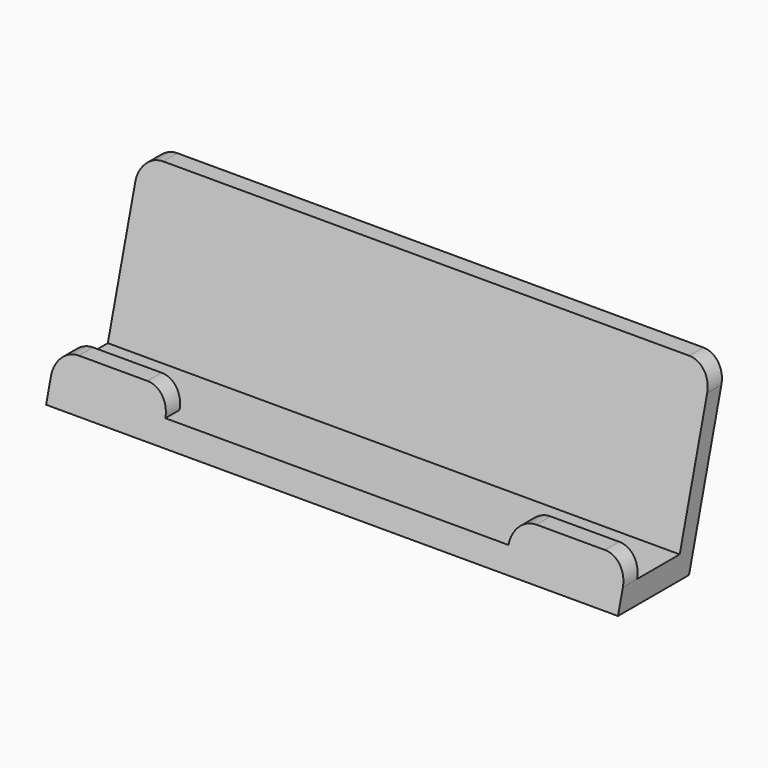
from build123d import *

# Parameters (mm, degrees)
F1_DEPTH = 100
F3_START = -45
F3_DEPTH = 10
F4_R     = 4
F5_W     = 60
F5_H     = 8.6717781019
F6_DEPTH = 4
F7_R     = 3.99999


# Not quite as in the source:
# - a fillet or chamfer is up to 0.001 mm smaller than in the source, because OpenCascade refuses the exact size


with BuildPart() as f1:
    # F0 (on Right) → F1 (new body)
    with BuildSketch(Plane.YZ):
        Polygon((-5.0582498297, 30.4073218231), (-8.1640783709, 30.4073218231), (-15.2398989277, 4), (-24.5573845514, 4), (-23.4855877816, 8), (-26.5914163229, 8), (-28.7350098623, 0), (-13.2058671562, 0), align=None)
    extrude(amount=F1_DEPTH)

    # F2 (on face) → F3 (join)
    with BuildSketch(Plane(origin=(0, 0, 0), x_dir=(0, -1, 0), z_dir=(-1, 0, 0)).offset(F3_START)):
        Polygon((13.2058671562, 0), (6.7691872092, 24.0220165943), (-22.3890729249, 3.8824980147), (-22.3890729249, 0), align=None)
    extrude(amount=-F3_DEPTH)

    # F4 (call 1 of 6: OpenCascade refuses the feature's edges together)
    f4_edges = [f1.edges().sort_by_distance(p)[0] for p in [
        (0, -6.611164, 30.407322),
    ]]
    fillet(f4_edges, radius=F4_R)

    # F4#2 (call 2 of 6)
    f4_2_edges = [f1.edges().sort_by_distance(p)[0] for p in [
        (100, -6.611164, 30.407322),
    ]]
    fillet(f4_2_edges, radius=F4_R)

    # F4#3 (call 3 of 6)
    f4_3_edges = [f1.edges().sort_by_distance(p)[0] for p in [
        (100, -25.038502, 8),
    ]]
    fillet(f4_3_edges, radius=F4_R)

    # F4#4 (call 4 of 6)
    f4_4_edges = [f1.edges().sort_by_distance(p)[0] for p in [
        (0, -25.038502, 8),
    ]]
    fillet(f4_4_edges, radius=F4_R)

    # F4#5 (call 5 of 6)
    f4_5_edges = [f1.edges().sort_by_distance(p)[0] for p in [
        (50, 22.389073, 3.882498),
    ]]
    fillet(f4_5_edges, radius=F4_R)

    # F4#6 (call 6 of 6)
    f4_6_edges = [f1.edges().sort_by_distance(p)[0] for p in [
        (50, -6.769187, 24.022017),
        (45, -9.987527, 12.011008),
        (55, -9.987527, 12.011008),
    ]]
    fillet(f4_6_edges, radius=F4_R)

    # F5 (on face) → F6 (cut)
    with BuildSketch(Plane.XY.offset(8)):
        with Locations((50, -27.8214768326)):
            Rectangle(F5_W, F5_H)
    extrude(amount=-F6_DEPTH, mode=Mode.SUBTRACT)

    # F7 (radius 4 in the source; OpenCascade refuses exactly that, so slightly less here)
    f7_edges = [f1.edges().sort_by_distance(p)[0] for p in [
        (20, -25.038502, 8),
        (80, -25.038502, 8),
    ]]
    fillet(f7_edges, radius=F7_R)


solid = f1.part
